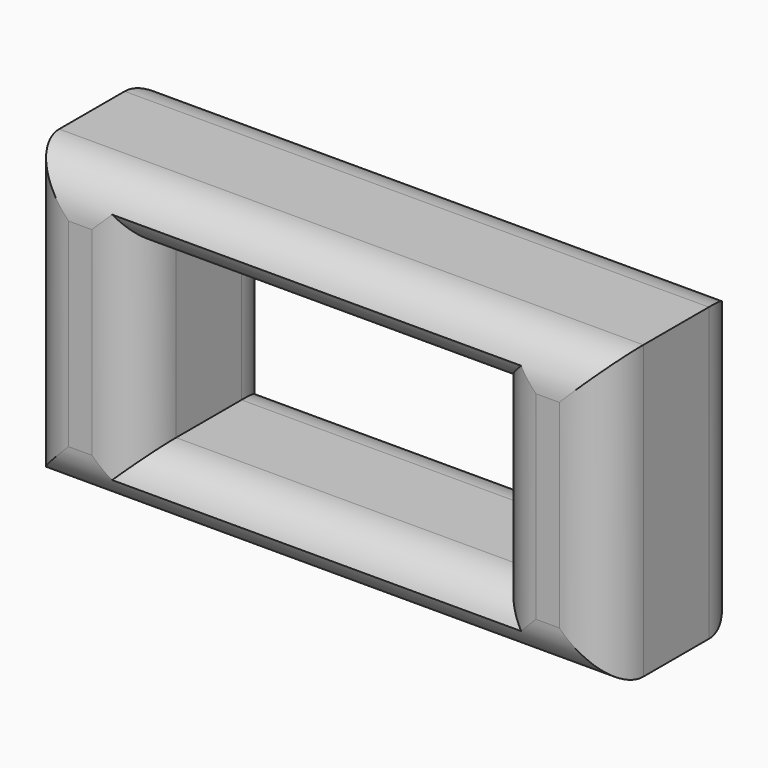
from build123d import *

# Parameters (mm, degrees)
F0_W          = 127
F0_H          = 63.5
F0_W_2        = 76.2
F0_H_2        = 38.1
F1_DEPTH      = 38.1
F2_T1_DEPTH   = 177.8
F2_T3_DEPTH   = 114.3
F2_T5_DEPTH   = 76.2
F2_T7_DEPTH   = 38.1
F2_T13_DEPTH  = 101.6
F2_T17_DEPTH  = 63.5
F2_T25_DEPTH  = 101.6
F2_T29_DEPTH  = 63.5
F2_T37_DEPTH  = 63.5
F2_T42_DEPTH  = 101.6
F2_T49_DEPTH  = 101.6
F2_T53_DEPTH  = 63.5
F2_T61_DEPTH  = 101.6
F2_T65_DEPTH  = 63.5
F2_T73_DEPTH  = 101.6
F2_T77_DEPTH  = 63.5
F2_T85_DEPTH  = 63.5
F2_T90_DEPTH  = 101.6
F2_T97_DEPTH  = 101.6
F2_T101_DEPTH = 63.5


# Not quite as in the source:
# - a fillet or chamfer that OpenCascade refuses, or shapes differently, is made with other operations: its cross-section is extruded or revolved along the edge and cut away or added


with BuildPart() as f1:
    # F0 (on Front) → F1 (new body)
    with BuildSketch(Plane.XZ):
        Rectangle(F0_W, F0_H)
        Rectangle(F0_W_2, F0_H_2, mode=Mode.SUBTRACT)
    extrude(amount=F1_DEPTH)

    # F2: fillet of radius 10.16 on 16 edges, made by hand

    # F2_s2 → F2_t1 (cut)
    with BuildSketch(Plane.YZ.offset(-88.9)):
        with BuildLine():
            ThreePointArc((-27.94, -31.75), (-35.1242048969, -28.7742048969), (-38.1, -21.59))
            Line((-38.1, -21.59), (-38.1, -31.75))
            Line((-38.1, -31.75), (-27.94, -31.75))
        make_face()
        with BuildLine():
            ThreePointArc((-27.94, 31.75), (-35.1242048969, 28.7742048969), (-38.1, 21.59))
            Line((-38.1, 21.59), (-38.1, 31.75))
            Line((-38.1, 31.75), (-27.94, 31.75))
        make_face()
        with BuildLine():
            ThreePointArc((-10.16, -31.75), (-2.9757951031, -28.7742048969), (0, -21.59))
            Line((0, -21.59), (0, -31.75))
            Line((0, -31.75), (-10.16, -31.75))
        make_face()
        with BuildLine():
            ThreePointArc((-10.16, 31.75), (-2.9757951031, 28.7742048969), (0, 21.59))
            Line((0, 21.59), (0, 31.75))
            Line((0, 31.75), (-10.16, 31.75))
        make_face()
    extrude(amount=F2_T1_DEPTH, mode=Mode.SUBTRACT)

    # F2_s4 → F2_t3 (cut)
    with BuildSketch(Plane.XY.offset(-57.15)):
        with BuildLine():
            ThreePointArc((63.5, -27.94), (60.5242048969, -35.1242048969), (53.34, -38.1))
            Line((53.34, -38.1), (63.5, -38.1))
            Line((63.5, -38.1), (63.5, -27.94))
        make_face()
        with BuildLine():
            ThreePointArc((-63.5, -27.94), (-60.5242048969, -35.1242048969), (-53.34, -38.1))
            Line((-53.34, -38.1), (-63.5, -38.1))
            Line((-63.5, -38.1), (-63.5, -27.94))
        make_face()
        with BuildLine():
            ThreePointArc((63.5, -10.16), (60.5242048969, -2.9757951031), (53.34, 0))
            Line((53.34, 0), (63.5, 0))
            Line((63.5, 0), (63.5, -10.16))
        make_face()
        with BuildLine():
            ThreePointArc((-63.5, -10.16), (-60.5242048969, -2.9757951031), (-53.34, 0))
            Line((-53.34, 0), (-63.5, 0))
            Line((-63.5, 0), (-63.5, -10.16))
        make_face()
    extrude(amount=F2_T3_DEPTH, mode=Mode.SUBTRACT)

    # F2_s6 → F2_t5 (cut)
    with BuildSketch(Plane.YZ.offset(-38.1)):
        with BuildLine():
            ThreePointArc((-27.94, -19.05), (-35.1242048969, -22.0257951031), (-38.1, -29.21))
            Line((-38.1, -29.21), (-38.1, -19.05))
            Line((-38.1, -19.05), (-27.94, -19.05))
        make_face()
        with BuildLine():
            ThreePointArc((-27.94, 19.05), (-35.1242048969, 22.0257951031), (-38.1, 29.21))
            Line((-38.1, 29.21), (-38.1, 19.05))
            Line((-38.1, 19.05), (-27.94, 19.05))
        make_face()
        with BuildLine():
            ThreePointArc((-10.16, -19.05), (-2.9757951031, -22.0257951031), (0, -29.21))
            Line((0, -29.21), (0, -19.05))
            Line((0, -19.05), (-10.16, -19.05))
        make_face()
        with BuildLine():
            ThreePointArc((-10.16, 19.05), (-2.9757951031, 22.0257951031), (0, 29.21))
            Line((0, 29.21), (0, 19.05))
            Line((0, 19.05), (-10.16, 19.05))
        make_face()
    extrude(amount=F2_T5_DEPTH, mode=Mode.SUBTRACT)

    # F2_s8 → F2_t7 (cut)
    with BuildSketch(Plane.XY.offset(-19.05)):
        with BuildLine():
            ThreePointArc((-38.1, -27.94), (-41.0757951031, -35.1242048969), (-48.26, -38.1))
            Line((-48.26, -38.1), (-38.1, -38.1))
            Line((-38.1, -38.1), (-38.1, -27.94))
        make_face()
        with BuildLine():
            ThreePointArc((38.1, -27.94), (41.0757951031, -35.1242048969), (48.26, -38.1))
            Line((48.26, -38.1), (38.1, -38.1))
            Line((38.1, -38.1), (38.1, -27.94))
        make_face()
        with BuildLine():
            ThreePointArc((-38.1, -10.16), (-41.0757951031, -2.9757951031), (-48.26, 0))
            Line((-48.26, 0), (-38.1, 0))
            Line((-38.1, 0), (-38.1, -10.16))
        make_face()
        with BuildLine():
            ThreePointArc((38.1, -10.16), (41.0757951031, -2.9757951031), (48.26, 0))
            Line((48.26, 0), (38.1, 0))
            Line((38.1, 0), (38.1, -10.16))
        make_face()
    extrude(amount=F2_T7_DEPTH, mode=Mode.SUBTRACT)


with BuildPart() as f2_tool11:
    # F2_s12 → F2_t13 (new body)
    with BuildSketch(Plane.YZ.offset(63.5)):
        with BuildLine():
            ThreePointArc((-27.94, -19.05), (-35.1242048969, -22.0257951031), (-38.1, -29.21))
            Line((-38.1, -29.21), (-38.1, -19.05))
            Line((-38.1, -19.05), (-27.94, -19.05))
        make_face()
    extrude(amount=-F2_T13_DEPTH)

    split(bisect_by=Plane.YZ.offset(38.1), keep=Keep.TOP)


with BuildPart() as f2_tool15:
    # F2_s16 → F2_t17 (new body)
    with BuildSketch(Plane.XY.offset(19.05)):
        with BuildLine():
            ThreePointArc((38.1, -27.94), (41.0757951031, -35.1242048969), (48.26, -38.1))
            Line((48.26, -38.1), (38.1, -38.1))
            Line((38.1, -38.1), (38.1, -27.94))
        make_face()
    extrude(amount=-F2_T17_DEPTH)

    split(bisect_by=Plane.XY.offset(-31.75), keep=Keep.TOP)

    split(bisect_by=Plane.XY.offset(-19.05), keep=Keep.BOTTOM)


with BuildPart() as f2_tool11_1:
    add(f2_tool11.part)

    # F2_t20: intersect F2_tool15
    add(f2_tool15.part, mode=Mode.INTERSECT)


with BuildPart() as f1_1:
    add(f1.part)

    # F2_t9: cut F2_tool11
    add(f2_tool11_1.part, mode=Mode.SUBTRACT)


with BuildPart() as f2_tool23:
    # F2_s24 → F2_t25 (new body)
    with BuildSketch(Plane.YZ.offset(38.1)):
        with BuildLine():
            ThreePointArc((-27.94, -19.05), (-35.1242048969, -22.0257951031), (-38.1, -29.21))
            Line((-38.1, -29.21), (-38.1, -19.05))
            Line((-38.1, -19.05), (-27.94, -19.05))
        make_face()
    extrude(amount=-F2_T25_DEPTH)

    split(bisect_by=Plane.YZ.offset(-38.1), keep=Keep.BOTTOM)


with BuildPart() as f2_tool27:
    # F2_s28 → F2_t29 (new body)
    with BuildSketch(Plane.XY.offset(-44.45)):
        with BuildLine():
            ThreePointArc((-38.1, -27.94), (-41.0757951031, -35.1242048969), (-48.26, -38.1))
            Line((-48.26, -38.1), (-38.1, -38.1))
            Line((-38.1, -38.1), (-38.1, -27.94))
        make_face()
    extrude(amount=F2_T29_DEPTH)

    split(bisect_by=Plane.XY.offset(-31.75), keep=Keep.TOP)

    split(bisect_by=Plane.XY.offset(-19.05), keep=Keep.BOTTOM)


with BuildPart() as f2_tool23_1:
    add(f2_tool23.part)

    # F2_t32: intersect F2_tool27
    add(f2_tool27.part, mode=Mode.INTERSECT)


with BuildPart() as f1_2:
    add(f1_1.part)

    # F2_t21: cut F2_tool23
    add(f2_tool23_1.part, mode=Mode.SUBTRACT)


with BuildPart() as f2_tool35:
    # F2_s36 → F2_t37 (new body)
    with BuildSketch(Plane.XY.offset(-19.05)):
        with BuildLine():
            ThreePointArc((-38.1, -27.94), (-41.0757951031, -35.1242048969), (-48.26, -38.1))
            Line((-48.26, -38.1), (-38.1, -38.1))
            Line((-38.1, -38.1), (-38.1, -27.94))
        make_face()
    extrude(amount=F2_T37_DEPTH)

    split(bisect_by=Plane.XY.offset(31.75), keep=Keep.BOTTOM)

    split(bisect_by=Plane.XY.offset(19.05), keep=Keep.TOP)


with BuildPart() as f2_tool40:
    # F2_s41 → F2_t42 (new body)
    with BuildSketch(Plane.YZ.offset(-63.5)):
        with BuildLine():
            ThreePointArc((-27.94, 19.05), (-35.1242048969, 22.0257951031), (-38.1, 29.21))
            Line((-38.1, 29.21), (-38.1, 19.05))
            Line((-38.1, 19.05), (-27.94, 19.05))
        make_face()
    extrude(amount=F2_T42_DEPTH)

    split(bisect_by=Plane.YZ.offset(-38.1), keep=Keep.BOTTOM)


with BuildPart() as f2_tool35_1:
    add(f2_tool35.part)

    # F2_t44: intersect F2_tool40
    add(f2_tool40.part, mode=Mode.INTERSECT)


with BuildPart() as f1_3:
    add(f1_2.part)

    # F2_t33: cut F2_tool35
    add(f2_tool35_1.part, mode=Mode.SUBTRACT)


with BuildPart() as f2_tool47:
    # F2_s48 → F2_t49 (new body)
    with BuildSketch(Plane.YZ.offset(-38.1)):
        with BuildLine():
            ThreePointArc((-27.94, 19.05), (-35.1242048969, 22.0257951031), (-38.1, 29.21))
            Line((-38.1, 29.21), (-38.1, 19.05))
            Line((-38.1, 19.05), (-27.94, 19.05))
        make_face()
    extrude(amount=F2_T49_DEPTH)

    split(bisect_by=Plane.YZ.offset(38.1), keep=Keep.TOP)


with BuildPart() as f2_tool51:
    # F2_s52 → F2_t53 (new body)
    with BuildSketch(Plane.XY.offset(44.45)):
        with BuildLine():
            ThreePointArc((38.1, -27.94), (41.0757951031, -35.1242048969), (48.26, -38.1))
            Line((48.26, -38.1), (38.1, -38.1))
            Line((38.1, -38.1), (38.1, -27.94))
        make_face()
    extrude(amount=-F2_T53_DEPTH)

    split(bisect_by=Plane.XY.offset(31.75), keep=Keep.BOTTOM)

    split(bisect_by=Plane.XY.offset(19.05), keep=Keep.TOP)


with BuildPart() as f2_tool47_1:
    add(f2_tool47.part)

    # F2_t56: intersect F2_tool51
    add(f2_tool51.part, mode=Mode.INTERSECT)


with BuildPart() as f1_4:
    add(f1_3.part)

    # F2_t45: cut F2_tool47
    add(f2_tool47_1.part, mode=Mode.SUBTRACT)


with BuildPart() as f2_tool59:
    # F2_s60 → F2_t61 (new body)
    with BuildSketch(Plane.YZ.offset(63.5)):
        with BuildLine():
            ThreePointArc((-10.16, -19.05), (-2.9757951031, -22.0257951031), (0, -29.21))
            Line((0, -29.21), (0, -19.05))
            Line((0, -19.05), (-10.16, -19.05))
        make_face()
    extrude(amount=-F2_T61_DEPTH)

    split(bisect_by=Plane.YZ.offset(38.1), keep=Keep.TOP)


with BuildPart() as f2_tool63:
    # F2_s64 → F2_t65 (new body)
    with BuildSketch(Plane.XY.offset(19.05)):
        with BuildLine():
            ThreePointArc((38.1, -10.16), (41.0757951031, -2.9757951031), (48.26, 0))
            Line((48.26, 0), (38.1, 0))
            Line((38.1, 0), (38.1, -10.16))
        make_face()
    extrude(amount=-F2_T65_DEPTH)

    split(bisect_by=Plane.XY.offset(-31.75), keep=Keep.TOP)

    split(bisect_by=Plane.XY.offset(-19.05), keep=Keep.BOTTOM)


with BuildPart() as f2_tool59_1:
    add(f2_tool59.part)

    # F2_t68: intersect F2_tool63
    add(f2_tool63.part, mode=Mode.INTERSECT)


with BuildPart() as f1_5:
    add(f1_4.part)

    # F2_t57: cut F2_tool59
    add(f2_tool59_1.part, mode=Mode.SUBTRACT)


with BuildPart() as f2_tool71:
    # F2_s72 → F2_t73 (new body)
    with BuildSketch(Plane.YZ.offset(38.1)):
        with BuildLine():
            ThreePointArc((-10.16, -19.05), (-2.9757951031, -22.0257951031), (0, -29.21))
            Line((0, -29.21), (0, -19.05))
            Line((0, -19.05), (-10.16, -19.05))
        make_face()
    extrude(amount=-F2_T73_DEPTH)

    split(bisect_by=Plane.YZ.offset(-38.1), keep=Keep.BOTTOM)


with BuildPart() as f2_tool75:
    # F2_s76 → F2_t77 (new body)
    with BuildSketch(Plane.XY.offset(-44.45)):
        with BuildLine():
            ThreePointArc((-38.1, -10.16), (-41.0757951031, -2.9757951031), (-48.26, 0))
            Line((-48.26, 0), (-38.1, 0))
            Line((-38.1, 0), (-38.1, -10.16))
        make_face()
    extrude(amount=F2_T77_DEPTH)

    split(bisect_by=Plane.XY.offset(-31.75), keep=Keep.TOP)

    split(bisect_by=Plane.XY.offset(-19.05), keep=Keep.BOTTOM)


with BuildPart() as f2_tool71_1:
    add(f2_tool71.part)

    # F2_t80: intersect F2_tool75
    add(f2_tool75.part, mode=Mode.INTERSECT)


with BuildPart() as f1_6:
    add(f1_5.part)

    # F2_t69: cut F2_tool71
    add(f2_tool71_1.part, mode=Mode.SUBTRACT)


with BuildPart() as f2_tool83:
    # F2_s84 → F2_t85 (new body)
    with BuildSketch(Plane.XY.offset(-19.05)):
        with BuildLine():
            ThreePointArc((-38.1, -10.16), (-41.0757951031, -2.9757951031), (-48.26, 0))
            Line((-48.26, 0), (-38.1, 0))
            Line((-38.1, 0), (-38.1, -10.16))
        make_face()
    extrude(amount=F2_T85_DEPTH)

    split(bisect_by=Plane.XY.offset(31.75), keep=Keep.BOTTOM)

    split(bisect_by=Plane.XY.offset(19.05), keep=Keep.TOP)


with BuildPart() as f2_tool88:
    # F2_s89 → F2_t90 (new body)
    with BuildSketch(Plane.YZ.offset(-63.5)):
        with BuildLine():
            ThreePointArc((-10.16, 19.05), (-2.9757951031, 22.0257951031), (0, 29.21))
            Line((0, 29.21), (0, 19.05))
            Line((0, 19.05), (-10.16, 19.05))
        make_face()
    extrude(amount=F2_T90_DEPTH)

    split(bisect_by=Plane.YZ.offset(-38.1), keep=Keep.BOTTOM)


with BuildPart() as f2_tool83_1:
    add(f2_tool83.part)

    # F2_t92: intersect F2_tool88
    add(f2_tool88.part, mode=Mode.INTERSECT)


with BuildPart() as f1_7:
    add(f1_6.part)

    # F2_t81: cut F2_tool83
    add(f2_tool83_1.part, mode=Mode.SUBTRACT)


with BuildPart() as f2_tool95:
    # F2_s96 → F2_t97 (new body)
    with BuildSketch(Plane.YZ.offset(-38.1)):
        with BuildLine():
            ThreePointArc((-10.16, 19.05), (-2.9757951031, 22.0257951031), (0, 29.21))
            Line((0, 29.21), (0, 19.05))
            Line((0, 19.05), (-10.16, 19.05))
        make_face()
    extrude(amount=F2_T97_DEPTH)

    split(bisect_by=Plane.YZ.offset(38.1), keep=Keep.TOP)


with BuildPart() as f2_tool99:
    # F2_s100 → F2_t101 (new body)
    with BuildSketch(Plane.XY.offset(44.45)):
        with BuildLine():
            ThreePointArc((38.1, -10.16), (41.0757951031, -2.9757951031), (48.26, 0))
            Line((48.26, 0), (38.1, 0))
            Line((38.1, 0), (38.1, -10.16))
        make_face()
    extrude(amount=-F2_T101_DEPTH)

    split(bisect_by=Plane.XY.offset(31.75), keep=Keep.BOTTOM)

    split(bisect_by=Plane.XY.offset(19.05), keep=Keep.TOP)


with BuildPart() as f2_tool95_1:
    add(f2_tool95.part)

    # F2_t104: intersect F2_tool99
    add(f2_tool99.part, mode=Mode.INTERSECT)


with BuildPart() as f1_8:
    add(f1_7.part)

    # F2_t93: cut F2_tool95
    add(f2_tool95_1.part, mode=Mode.SUBTRACT)


solid = f1_8.part
